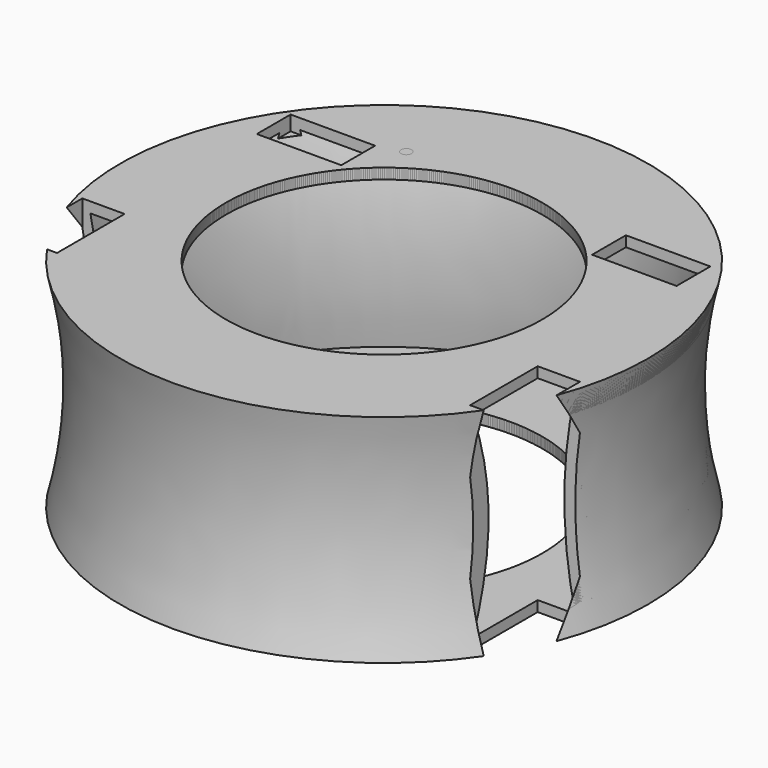
from build123d import *

# Parameters (mm, degrees)
F2_T      = -1.27
F4_D      = 1.27
F4_DEPTH  = 5.08
F4_TIP    = 0.3815464931
F5_COUNT  = 11
F6_W      = 10.16
F6_H      = 5.08
F7_DEPTH  = 1.778
F8_W      = 10.16
F8_H      = 5.0799990049
F9_DEPTH  = 1.778
F11_DEPTH = 26.035


with BuildPart() as f1:
    # F0 (on Front) → F1 (revolve)
    with BuildSketch(Plane.XZ):
        with BuildLine():
            ThreePointArc((-60.2397024632, 38.6090278625), (-58.6273197833, 25.5915278625), (-60.2397024632, 12.5740278625))
            Line((-60.2397024632, 12.5740278625), (-47.5397024632, 12.5740278625))
            Line((-47.5397024632, 12.5740278625), (-47.5397024632, 38.6090278625))
            Line((-47.5397024632, 38.6090278625), (-60.2397024632, 38.6090278625))
        make_face()
    revolve(axis=Axis((-28.491001968, 0, 25.3042703682), (0, 0, -1)))

    # F2
    f2_openings = [f1.faces().sort_by_distance(p)[0] for p in [
        (-9.442301, 0, 25.591528),
    ]]
    offset(amount=F2_T, openings=f2_openings)

    # F4
    with Locations(Plane.XY.offset(38.6090278625)):
        with Locations((-28.7121385336, 22.3573299974)):
            Hole(F4_D / 2, depth=F4_DEPTH)
            with Locations((0, 0, -(F4_DEPTH + F4_TIP / 2))):  # 118° drill point
                Cone(0, F4_D / 2, F4_TIP, mode=Mode.SUBTRACT)


with BuildPart() as f5_1:
    # F5: instance of F1
    add(f1.part.rotate(Axis((-28.491001968, 0, 38.6090278625), (0, 0, -1)), 1 * 360 / F5_COUNT))


with BuildPart() as f5_2:
    # F5: instance of F1
    add(f1.part.rotate(Axis((-28.491001968, 0, 38.6090278625), (0, 0, -1)), 2 * 360 / F5_COUNT))


with BuildPart() as f5_3:
    # F5: instance of F1
    add(f1.part.rotate(Axis((-28.491001968, 0, 38.6090278625), (0, 0, -1)), 3 * 360 / F5_COUNT))


with BuildPart() as f5_4:
    # F5: instance of F1
    add(f1.part.rotate(Axis((-28.491001968, 0, 38.6090278625), (0, 0, -1)), 4 * 360 / F5_COUNT))


with BuildPart() as f5_5:
    # F5: instance of F1
    add(f1.part.rotate(Axis((-28.491001968, 0, 38.6090278625), (0, 0, -1)), 5 * 360 / F5_COUNT))


with BuildPart() as f5_6:
    # F5: instance of F1
    add(f1.part.rotate(Axis((-28.491001968, 0, 38.6090278625), (0, 0, -1)), 6 * 360 / F5_COUNT))


with BuildPart() as f5_7:
    # F5: instance of F1
    add(f1.part.rotate(Axis((-28.491001968, 0, 38.6090278625), (0, 0, -1)), 7 * 360 / F5_COUNT))


with BuildPart() as f5_8:
    # F5: instance of F1
    add(f1.part.rotate(Axis((-28.491001968, 0, 38.6090278625), (0, 0, -1)), 8 * 360 / F5_COUNT))


with BuildPart() as f5_9:
    # F5: instance of F1
    add(f1.part.rotate(Axis((-28.491001968, 0, 38.6090278625), (0, 0, -1)), 9 * 360 / F5_COUNT))


with BuildPart() as f5_10:
    # F5: instance of F1
    add(f1.part.rotate(Axis((-28.491001968, 0, 38.6090278625), (0, 0, -1)), 10 * 360 / F5_COUNT))


with BuildPart() as f7_tool:
    # F6 (on face) → F7 (new body)
    with BuildSketch(Plane.XY.offset(38.6090278625)):
        with Locations((-8.9602516699, 15.7516787136)):
            Rectangle(F6_W, F6_H)
    extrude(amount=-F7_DEPTH)


with BuildPart() as f1_1:
    add(f1.part)

    # F7: cut by f7_tool
    add(f7_tool.part, mode=Mode.SUBTRACT)


with BuildPart() as f5_1_1:
    add(f5_1.part)

    # F7: cut by f7_tool
    add(f7_tool.part, mode=Mode.SUBTRACT)


with BuildPart() as f5_2_1:
    add(f5_2.part)

    # F7: cut by f7_tool
    add(f7_tool.part, mode=Mode.SUBTRACT)


with BuildPart() as f5_3_1:
    add(f5_3.part)

    # F7: cut by f7_tool
    add(f7_tool.part, mode=Mode.SUBTRACT)


with BuildPart() as f5_4_1:
    add(f5_4.part)

    # F7: cut by f7_tool
    add(f7_tool.part, mode=Mode.SUBTRACT)


with BuildPart() as f5_5_1:
    add(f5_5.part)

    # F7: cut by f7_tool
    add(f7_tool.part, mode=Mode.SUBTRACT)


with BuildPart() as f5_6_1:
    add(f5_6.part)

    # F7: cut by f7_tool
    add(f7_tool.part, mode=Mode.SUBTRACT)


with BuildPart() as f5_7_1:
    add(f5_7.part)

    # F7: cut by f7_tool
    add(f7_tool.part, mode=Mode.SUBTRACT)


with BuildPart() as f5_8_1:
    add(f5_8.part)

    # F7: cut by f7_tool
    add(f7_tool.part, mode=Mode.SUBTRACT)


with BuildPart() as f5_9_1:
    add(f5_9.part)

    # F7: cut by f7_tool
    add(f7_tool.part, mode=Mode.SUBTRACT)


with BuildPart() as f5_10_1:
    add(f5_10.part)

    # F7: cut by f7_tool
    add(f7_tool.part, mode=Mode.SUBTRACT)


with BuildPart() as f9_tool:
    # F8 (on face) → F9 (new body)
    with BuildSketch(Plane.XY.offset(38.6090278625)):
        with Locations((-48.8920975477, 15.2571792714)):
            Rectangle(F8_W, F8_H)
    extrude(amount=-F9_DEPTH)


with BuildPart() as f1_2:
    add(f1_1.part)

    # F9: cut by f9_tool
    add(f9_tool.part, mode=Mode.SUBTRACT)


with BuildPart() as f5_1_2:
    add(f5_1_1.part)

    # F9: cut by f9_tool
    add(f9_tool.part, mode=Mode.SUBTRACT)


with BuildPart() as f5_2_2:
    add(f5_2_1.part)

    # F9: cut by f9_tool
    add(f9_tool.part, mode=Mode.SUBTRACT)


with BuildPart() as f5_3_2:
    add(f5_3_1.part)

    # F9: cut by f9_tool
    add(f9_tool.part, mode=Mode.SUBTRACT)


with BuildPart() as f5_4_2:
    add(f5_4_1.part)

    # F9: cut by f9_tool
    add(f9_tool.part, mode=Mode.SUBTRACT)


with BuildPart() as f5_5_2:
    add(f5_5_1.part)

    # F9: cut by f9_tool
    add(f9_tool.part, mode=Mode.SUBTRACT)


with BuildPart() as f5_6_2:
    add(f5_6_1.part)

    # F9: cut by f9_tool
    add(f9_tool.part, mode=Mode.SUBTRACT)


with BuildPart() as f5_7_2:
    add(f5_7_1.part)

    # F9: cut by f9_tool
    add(f9_tool.part, mode=Mode.SUBTRACT)


with BuildPart() as f5_8_2:
    add(f5_8_1.part)

    # F9: cut by f9_tool
    add(f9_tool.part, mode=Mode.SUBTRACT)


with BuildPart() as f5_9_2:
    add(f5_9_1.part)

    # F9: cut by f9_tool
    add(f9_tool.part, mode=Mode.SUBTRACT)


with BuildPart() as f5_10_2:
    add(f5_10_1.part)

    # F9: cut by f9_tool
    add(f9_tool.part, mode=Mode.SUBTRACT)


with BuildPart() as f11_tool:
    # F10 (on face) → F11 (new body)
    with BuildSketch(Plane.XY.offset(38.6090278625)):
        with BuildLine():
            Line((-53.5090583766, -7.7422231596), (-58.5890583766, -7.7422231596))
            Line((-58.5890583766, -7.7422231596), (-58.5890583766, -10.1038103485))
            ThreePointArc((-58.5890583766, -10.1038103485), (-56.9187304753, -14.1366274282), (-54.7110398984, -17.9022231596))
            Line((-54.7110398984, -17.9022231596), (-53.5090583766, -17.9022231596))
            Line((-53.5090583766, -17.9022231596), (-53.5090583766, -7.7422231596))
        make_face()
        with BuildLine():
            ThreePointArc((-54.7110398984, -17.9022231596), (-56.9187304753, -14.1366274282), (-58.5890583766, -10.1038103485))
            Line((-58.5890583766, -10.1038103485), (-58.5890583766, -17.9022231596))
            Line((-58.5890583766, -17.9022231596), (-54.7110398984, -17.9022231596))
        make_face()
        with BuildLine():
            ThreePointArc((-2.2305042536, -17.8428204868), (-0.3124506617, -14.6270034324), (1.2136558495, -11.2077333605))
            Line((1.2136558495, -11.2077333605), (1.2136558495, -7.6828204868))
            Line((1.2136558495, -7.6828204868), (-3.8663441505, -7.6828204868))
            Line((-3.8663441505, -7.6828204868), (-3.8663441505, -17.8428204868))
            Line((-3.8663441505, -17.8428204868), (-2.2305042536, -17.8428204868))
        make_face()
        with BuildLine():
            Line((1.2136558495, -17.8428204868), (1.2136558495, -11.2077333605))
            ThreePointArc((1.2136558495, -11.2077333605), (-0.3124506617, -14.6270034324), (-2.2305042536, -17.8428204868))
            Line((-2.2305042536, -17.8428204868), (1.2136558495, -17.8428204868))
        make_face()
    extrude(amount=-F11_DEPTH)


with BuildPart() as f1_3:
    add(f1_2.part)

    # F11: cut by f11_tool
    add(f11_tool.part, mode=Mode.SUBTRACT)


with BuildPart() as f5_1_3:
    add(f5_1_2.part)

    # F11: cut by f11_tool
    add(f11_tool.part, mode=Mode.SUBTRACT)


with BuildPart() as f5_2_3:
    add(f5_2_2.part)

    # F11: cut by f11_tool
    add(f11_tool.part, mode=Mode.SUBTRACT)


with BuildPart() as f5_3_3:
    add(f5_3_2.part)

    # F11: cut by f11_tool
    add(f11_tool.part, mode=Mode.SUBTRACT)


with BuildPart() as f5_4_3:
    add(f5_4_2.part)

    # F11: cut by f11_tool
    add(f11_tool.part, mode=Mode.SUBTRACT)


with BuildPart() as f5_5_3:
    add(f5_5_2.part)

    # F11: cut by f11_tool
    add(f11_tool.part, mode=Mode.SUBTRACT)


with BuildPart() as f5_6_3:
    add(f5_6_2.part)

    # F11: cut by f11_tool
    add(f11_tool.part, mode=Mode.SUBTRACT)


with BuildPart() as f5_7_3:
    add(f5_7_2.part)

    # F11: cut by f11_tool
    add(f11_tool.part, mode=Mode.SUBTRACT)


with BuildPart() as f5_8_3:
    add(f5_8_2.part)

    # F11: cut by f11_tool
    add(f11_tool.part, mode=Mode.SUBTRACT)


with BuildPart() as f5_9_3:
    add(f5_9_2.part)

    # F11: cut by f11_tool
    add(f11_tool.part, mode=Mode.SUBTRACT)


with BuildPart() as f5_10_3:
    add(f5_10_2.part)

    # F11: cut by f11_tool
    add(f11_tool.part, mode=Mode.SUBTRACT)


solid = Compound([f1_3.part, f5_1_3.part, f5_2_3.part, f5_3_3.part, f5_4_3.part, f5_5_3.part, f5_6_3.part, f5_7_3.part, f5_8_3.part, f5_9_3.part, f5_10_3.part])
